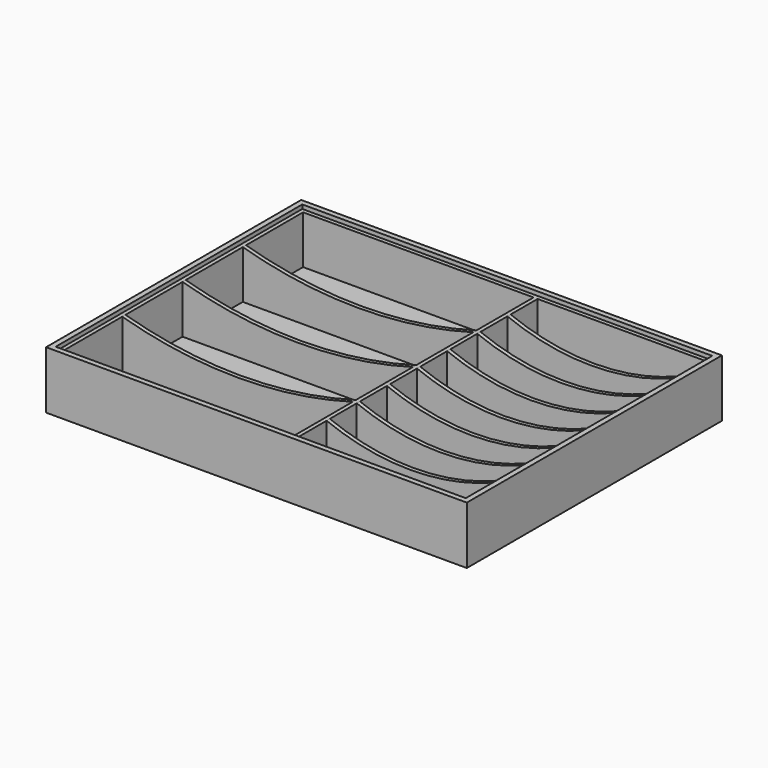
from build123d import *

# Parameters (mm, degrees)
F0_W     = 485.775
F0_H     = 365.125
F0_W_2   = 273.05
F0_H_2   = 87.8133544401
F0_H_3   = 84.4931
F0_W_3   = 198.4375
F0_H_4   = 43.1855544401
F0_H_5   = 39.8653
F0_H_6   = 84.5129455599
F0_H_7   = 39.8851455599
F1_DEPTH = 57.15
F0_W_4   = 498.475
F0_H_8   = 377.825
F2_DEPTH = 61.9125
F5_DEPTH = 315.7148544401
F3_W     = 498.475
F3_H     = 377.825
F6_DEPTH = 6.35


with BuildPart() as f1:
    # F0 (on Top) → F1 (new body)
    with BuildSketch(Plane.XY):
        with Locations((-7.6289700516, 36.4935102986)):
            Rectangle(F0_W, F0_H)
        with Locations((-109.2289700516, -97.3998124813)):
            Rectangle(F0_W_2, F0_H_2, mode=Mode.SUBTRACT)
        with Locations((-109.2289700516, -6.4840852612)):
            Rectangle(F0_W_2, F0_H_3, mode=Mode.SUBTRACT)
        with Locations((131.2772799484, -119.7137124813)):
            Rectangle(F0_W_3, F0_H_4, mode=Mode.SUBTRACT)
        with Locations((131.2772799484, -73.4257852612)):
            Rectangle(F0_W_3, F0_H_5, mode=Mode.SUBTRACT)
        with Locations((131.2772799484, -28.7979852612)):
            Rectangle(F0_W_3, F0_H_5, mode=Mode.SUBTRACT)
        with Locations((131.2772799484, 15.8298147388)):
            Rectangle(F0_W_3, F0_H_5, mode=Mode.SUBTRACT)
        with Locations((-109.2289700516, 82.7715147388)):
            Rectangle(F0_W_2, F0_H_3, mode=Mode.SUBTRACT)
        with Locations((-109.2289700516, 172.0370375187)):
            Rectangle(F0_W_2, F0_H_6, mode=Mode.SUBTRACT)
        with Locations((131.2772799484, 60.4576147388)):
            Rectangle(F0_W_3, F0_H_5, mode=Mode.SUBTRACT)
        with Locations((131.2772799484, 105.0854147388)):
            Rectangle(F0_W_3, F0_H_5, mode=Mode.SUBTRACT)
        with Locations((131.2772799484, 149.7132147388)):
            Rectangle(F0_W_3, F0_H_5, mode=Mode.SUBTRACT)
        with Locations((131.2772799484, 194.3509375187)):
            Rectangle(F0_W_3, F0_H_7, mode=Mode.SUBTRACT)
    extrude(amount=F1_DEPTH)

    # F4 (on face) → F5 (cut, through all)
    with BuildSketch(Plane(origin=(0, -141.3064897014, 0), x_dir=(-1, 0, 0), z_dir=(0, 1, 0))):
        with BuildLine():
            Line((-32.0585299484, 57.15), (-230.4960299484, 57.15))
            ThreePointArc((-230.4960299484, 57.15), (-131.2772799484, 38.1), (-32.0585299484, 57.15))
        make_face()
        with BuildLine():
            ThreePointArc((-27.2960299484, 57.15), (109.2289700516, 38.1), (245.7539700516, 57.15))
            Line((245.7539700516, 57.15), (-27.2960299484, 57.15))
        make_face()
    extrude(amount=F5_DEPTH, mode=Mode.SUBTRACT)


with BuildPart() as f2:
    # F0 (on Top) → F2 (new body)
    with BuildSketch(Plane.XY):
        with Locations((-7.6289700516, 36.4935102986)):
            Rectangle(F0_W_4, F0_H_8)
        with Locations((-7.6289700516, 36.4935102986)):
            Rectangle(F0_W, F0_H, mode=Mode.SUBTRACT)
    extrude(amount=F2_DEPTH)

    # F3 (on face) → F6 (join)
    with BuildSketch(Plane.XY):
        with Locations((-7.6289700516, 36.4935102986)):
            Rectangle(F3_W, F3_H)
    extrude(amount=-F6_DEPTH)


solid = Compound([f1.part, f2.part])
